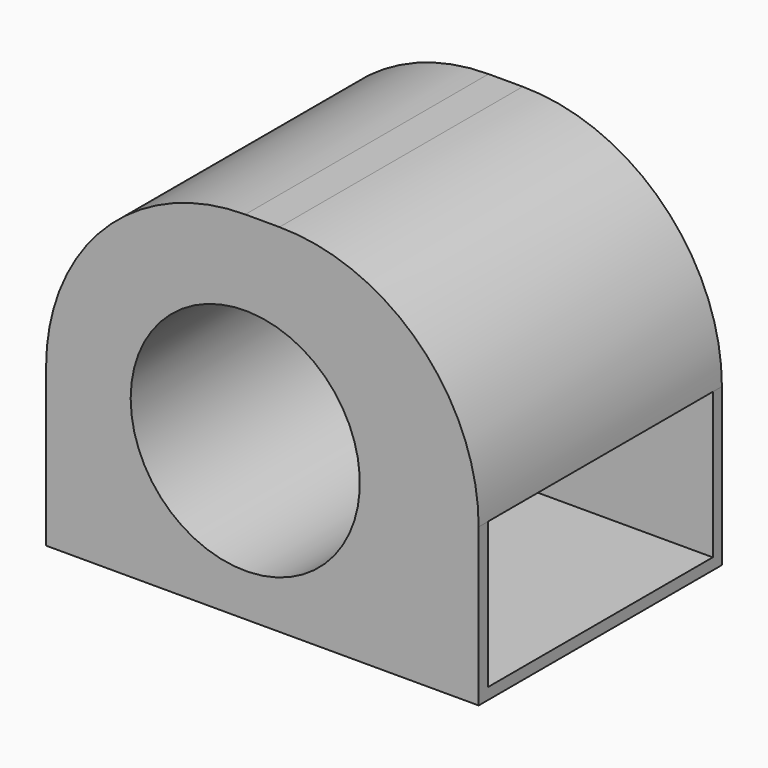
from build123d import *

# Parameters (mm, degrees)
F0_W     = 95.8885699511
F0_H     = 67.4029458314
F1_DEPTH = 78.994
F2_R     = 44.1511376287
F4_D     = 50.8
F5_T     = -2.54


# Not quite as in the source:
# - a shell that OpenCascade refuses in one call is made with other operations: the cavity is built on its own and cut out


with BuildPart() as f1:
    # F0 (on Top) → F1 (new body)
    with BuildSketch(Plane.XY):
        with Locations((-40.1296839118, -48.2643311843)):
            Rectangle(F0_W, F0_H)
    extrude(amount=F1_DEPTH)

    # F2
    f2_edges = [f1.edges().sort_by_distance(p)[0] for p in [
        (-88.073969, -48.264331, 78.994),
        (7.814601, -48.264331, 78.994),
    ]]
    fillet(f2_edges, radius=F2_R)

    # F4 (through all)
    with Locations(Plane.XZ.offset(81.9658041)):
        with Locations((-43.9228312586, 34.8428623713)):
            Hole(F4_D / 2)

    # F5: a shell. OpenCascade refuses it in one call, so the cavity is built on its own and cut out:
    # the body offset inwards by the wall thickness, plus a prism from it out through each open face.
    f5_core = offset(f1.part, amount=F5_T, mode=Mode.PRIVATE)
    f5_exits = [f5_core.faces().sort_by_distance(p)[0] for p in [
        (5.274601, -48.264331, 18.691431),
    ]]
    add(f5_core, mode=Mode.SUBTRACT)
    extrude(f5_exits, amount=-F5_T, mode=Mode.SUBTRACT)


solid = f1.part
